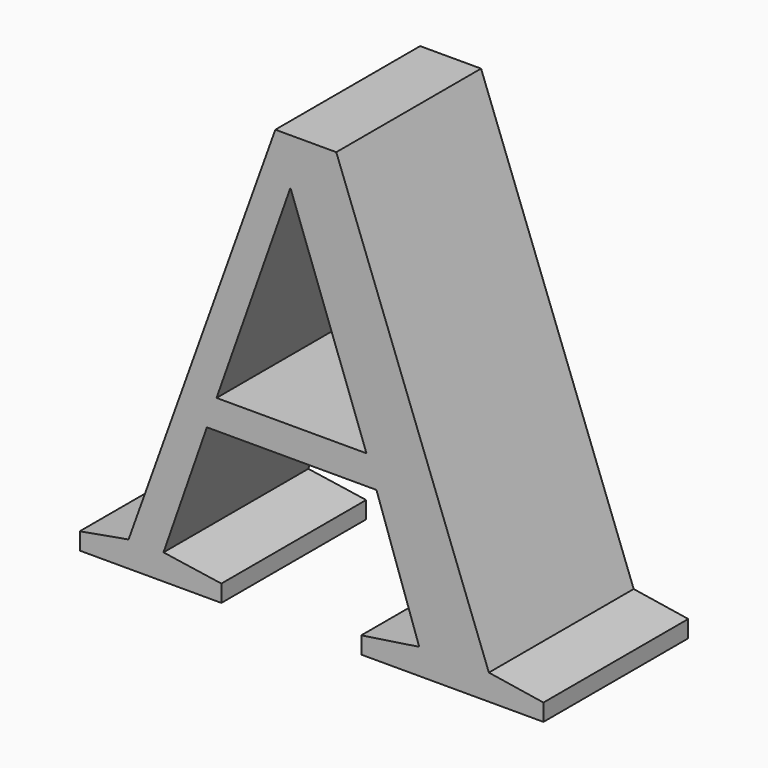
from build123d import *

# Parameters (mm, degrees)
F0_TEXT_SIZE = 46.1473750571
F1_DEPTH     = 12.7


# Not quite as in the source:
# - Text() gives the source's letters only with a copy of the font that has no kerning and outlines rounded to 1/6400 em; it was checked with that copy


with BuildPart() as f1:
    # F0 (on Front) → F1 (new body)
    with BuildSketch(Plane.XZ):
        with Locations((-46.4019812644, 3.246229142)):
            Text('A', F0_TEXT_SIZE, font='Tinos', text_align=(TextAlign.LEFT, TextAlign.BOTTOM))
    extrude(amount=F1_DEPTH)


solid = f1.part
